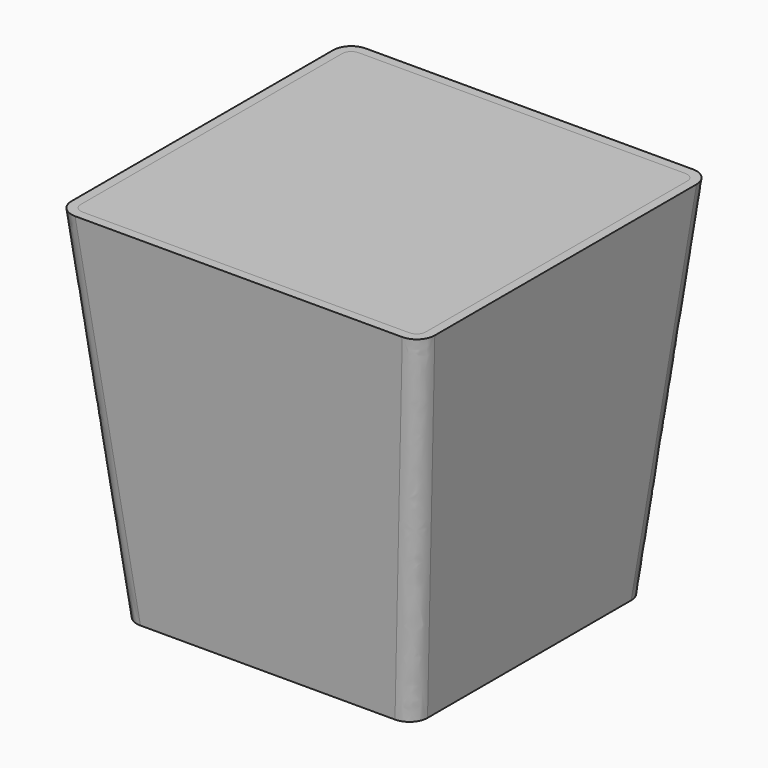
from build123d import *

# Parameters (mm, degrees)
F0_W      = 100
F0_H      = 100
F2_W      = 80
F2_H      = 80
F4_R      = 5
F5_T      = -2.5
F7_DEPTH  = 5
F8_R      = 1.5
F9_DEPTH  = 65.6
F10_DEPTH = 47.4875310947
F11_DEPTH = 47.4875310947


with BuildPart() as f3:
    # F0 (on Top) → F3 section 0
    with BuildSketch(Plane.XY):
        Rectangle(F0_W, F0_H)
    # F2 (on offset) → F3 section 1
    with BuildSketch(Plane.XY.offset(-100)):
        Rectangle(F2_W, F2_H)
    loft()

    # F4
    f4_edges = [f3.edges().sort_by_distance(p)[0] for p in [
        (45, 45, -50),
        (-45, 45, -50),
        (-45, -45, -50),
        (45, -45, -50),
    ]]
    fillet(f4_edges, radius=F4_R)

    # F5
    f5_openings = [f3.faces().sort_by_distance(p)[0] for p in [
        (0, 0, 0),
    ]]
    offset(amount=F5_T, openings=f5_openings, kind=Kind.INTERSECTION)


with BuildPart() as f7:
    # F6 (on Top) → F7 (new body)
    with BuildSketch(Plane.XY):
        with BuildLine():
            Line((-47.4875310947, 44.9999381192), (-47.4875310947, -44.9999381192))
            add(Edge.make_bspline(
                [(-47.4875310947, -44.9999381192), (-47.4875310947, -47.4875310947), (-44.9999381192, -47.4875310947)],
                knots=[5.5027377197, 5.5027377197, 5.5027377197, 7.0636328946, 7.0636328946, 7.0636328946], degree=2, weights=[1, 0.7105986878, 1]))
            Line((-44.9999381192, -47.4875310947), (44.9999381192, -47.4875310947))
            add(Edge.make_bspline(
                [(44.9999381192, -47.4875310947), (47.4875310947, -47.4875310947), (47.4875310947, -44.9999381192)],
                knots=[2.3611450661, 2.3611450661, 2.3611450661, 3.9220402411, 3.9220402411, 3.9220402411], degree=2, weights=[1, 0.7105986878, 1]))
            Line((47.4875310947, -44.9999381192), (47.4875310947, 44.9999381192))
            add(Edge.make_bspline(
                [(47.4875310947, 44.9999381192), (47.4875310947, 47.4875310947), (44.9999381192, 47.4875310947)],
                knots=[5.5027377197, 5.5027377197, 5.5027377197, 7.0636328946, 7.0636328946, 7.0636328946], degree=2, weights=[1, 0.7105986878, 1]))
            Line((44.9999381192, 47.4875310947), (-44.9999381192, 47.4875310947))
            add(Edge.make_bspline(
                [(-44.9999381192, 47.4875310947), (-47.4875310947, 47.4875310947), (-47.4875310947, 44.9999381192)],
                knots=[2.3611450661, 2.3611450661, 2.3611450661, 3.9220402411, 3.9220402411, 3.9220402411], degree=2, weights=[1, 0.7105986878, 1]))
        make_face()
    extrude(amount=-F7_DEPTH)

    # F8 (on Front) → F9 (cut, symmetric)
    with BuildSketch(Plane.XZ):
        with Locations((0, -2.5)):
            Circle(F8_R)
    extrude(amount=F9_DEPTH, both=True, mode=Mode.SUBTRACT)


with BuildPart() as f10:
    # F8 (on Front) → F10 (new body, through all)
    with BuildSketch(Plane.XZ):
        with Locations((0, -2.5)):
            Circle(F8_R)
    extrude(amount=F10_DEPTH)

    # F8 (on Front) → F11 (join, through all)
    with BuildSketch(Plane.XZ):
        with Locations((0, -2.5)):
            Circle(F8_R)
    extrude(amount=-F11_DEPTH)


solid = Compound([f3.part, f7.part, f10.part])
